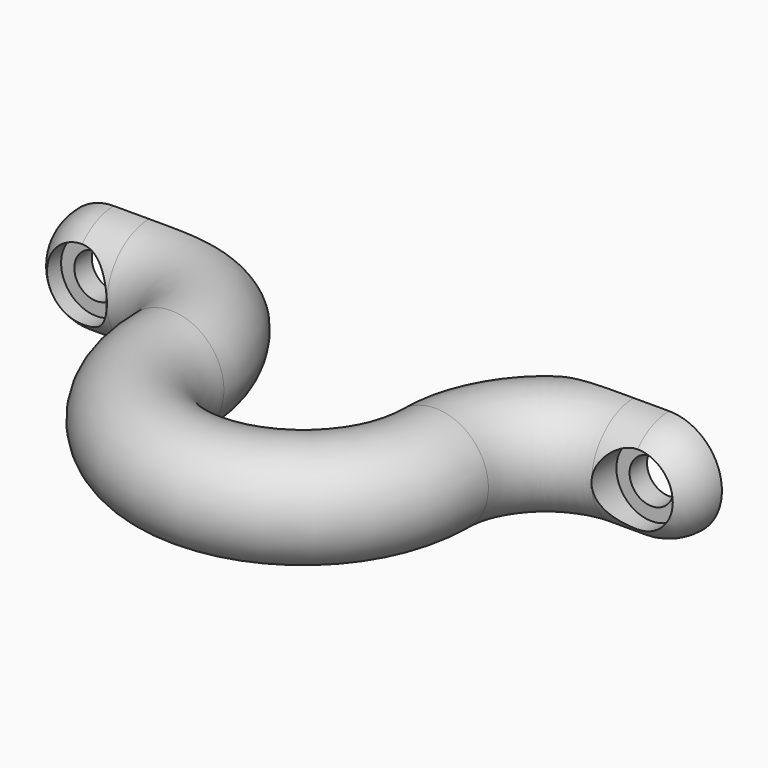
from build123d import *

# Parameters (mm, degrees)
F2_R            = 6
F4_DEPTH        = 10
F5_DEPTH        = 10
F9_W            = 85.8580678701
F9_H            = 17.2091361135
F10_DEPTH       = 25
F11_R           = 5.99999
F14_D           = 5
F14_START       = 1.5278641
F14_START_2     = 1.5278642
F14_CBORE_D     = 8
F14_CBORE_DEPTH = 2


# Not quite as in the source:
# - a fillet or chamfer is up to 0.001 mm smaller than in the source, because OpenCascade refuses the exact size


with BuildPart() as f3:
    # F3: sweep along a path in F0
    with BuildLine(Plane.XY) as f3_path:
        ThreePointArc((-27.5, 12.5), (-18.6611652352, 8.8388347648), (-15, 0))
        ThreePointArc((-15, 0), (0, -15), (15, 0))
        ThreePointArc((15, 0), (18.6611652352, 8.8388347648), (27.5, 12.5))
    # F2 (on offset) → F3 (sweep)
    with BuildSketch(Plane.YZ.offset(-27.5)):
        with Locations((12.5, 0)):
            Circle(F2_R)
    sweep(path=f3_path.line)

    # F4 (add): a face of the model
    f4_faces = [f3.faces().sort_by_distance(p)[0] for p in [
        (27.5, 12.5, 0),
    ]]
    extrude(f4_faces, amount=F4_DEPTH)

    # F5 (add): a face of the model
    f5_faces = [f3.faces().sort_by_distance(p)[0] for p in [
        (-27.5, 12.5, 0),
    ]]
    extrude(f5_faces, amount=F5_DEPTH)

    # F9 (on offset) → F10 (cut)
    with BuildSketch(Plane.XY.offset(6)):
        with Locations((5.4290339351, 21.1045680568)):
            Rectangle(F9_W, F9_H)
    extrude(amount=-F10_DEPTH, mode=Mode.SUBTRACT)

    # F11 (radius 6 in the source; OpenCascade refuses exactly that, so slightly less here)
    f11_edges = [f3.edges().sort_by_distance(p)[0] for p in [
        (-37.5, 6.5, 0),
        (37.5, 6.5, 0),
    ]]
    fillet(f11_edges, radius=F11_R)

    # F14 (through all)
    # its depths count from where the whole tool has entered the part; down to there all is cleared
    with Locations(Plane.XZ.offset(-6.5)):
        with Locations((-31.5, 0, -F14_START), (31.5, 6.2e-09, -F14_START_2)):
            CounterBoreHole(F14_D / 2, F14_CBORE_D / 2, F14_CBORE_DEPTH)


solid = f3.part
